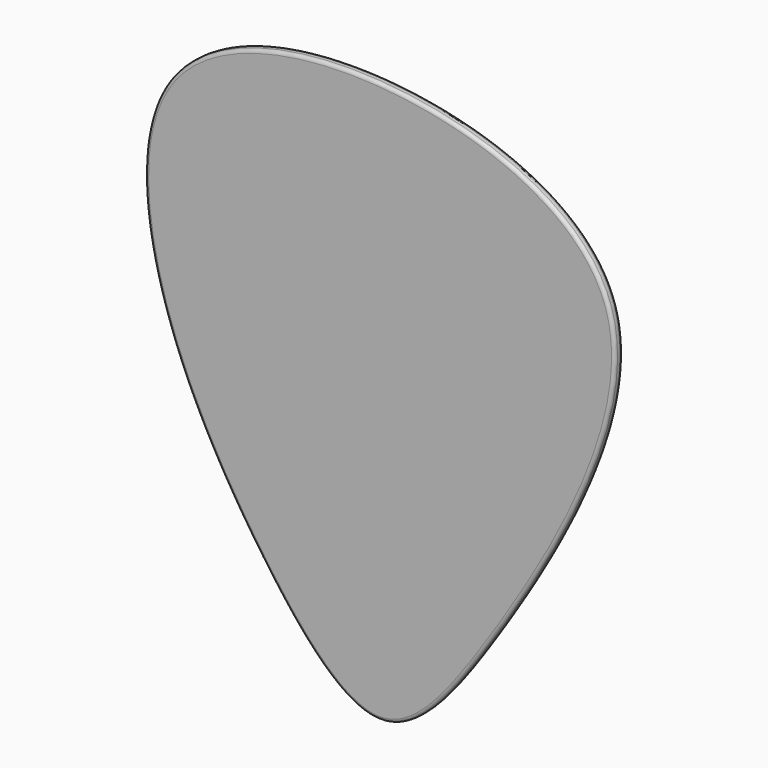
from build123d import *

# Parameters (mm, degrees)
F1_DEPTH = 0.88
F2_R     = 0.3


with BuildPart() as f1:
    # F0 (on Front) → F1 (new body)
    with BuildSketch(Plane.XZ):
        with BuildLine():
            add(Edge.make_bspline(
                [(0, 22.0081880689), (-8.028032589, 22.5679101346), (-21.8543308582, 19.0668708073), (-21.4852637626, -1.1721370581), (-11.3769871922, -19.4154320026), (0.3184544265, -33.0118724706), (10.988232546, -19.456997901), (30.2837691587, 13.7206458327), (8.8989956195, 21.3877416325), (0, 22.0081880689)],
                knots=[0, 0, 0, 0, 0.141614735, 0.2715972345, 0.4233724876, 0.541419927, 0.6610885531, 0.843021451, 1, 1, 1, 1], degree=3))
        make_face()
    extrude(amount=F1_DEPTH)

    # F2
    f2_edges = [f1.edges().sort_by_distance(p)[0] for p in [
        (-0.438485, -0.88, -28.968202),
        (-0.438485, 0, -28.968202),
    ]]
    fillet(f2_edges, radius=F2_R)


solid = f1.part
